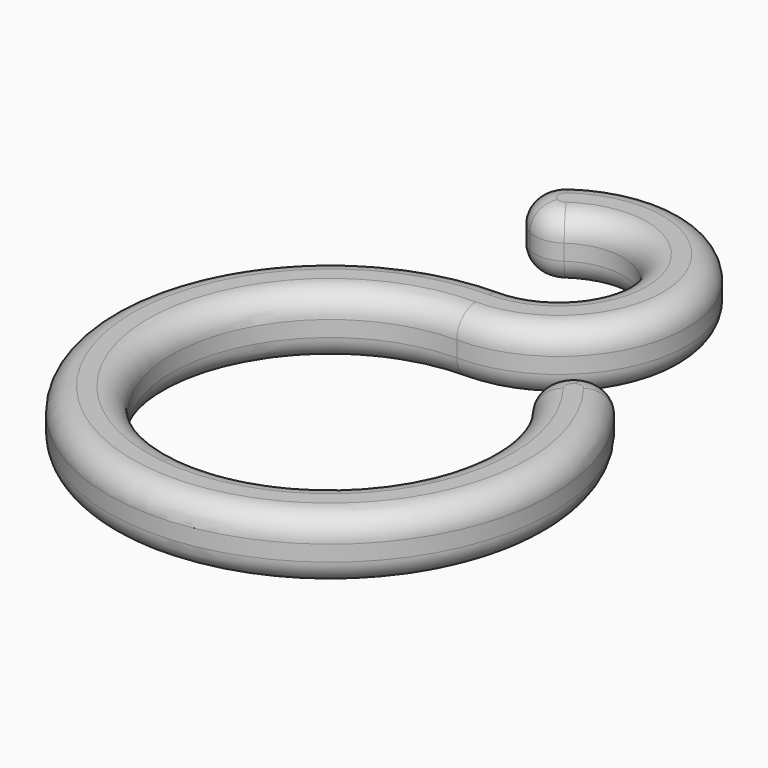
from build123d import *

# Parameters (mm, degrees)
F1_DEPTH = 4
F2_R     = 1.99999
F3_R     = 1.5


# Not quite as in the source:
# - a fillet or chamfer is up to 0.001 mm smaller than in the source, because OpenCascade refuses the exact size


with BuildPart() as f1:
    # F0 (on Top) → F1 (new body)
    with BuildSketch(Plane.XY):
        with BuildLine():
            ThreePointArc((-6.4063729182, 27.757124237), (0.3935028475, 26.9429632102), (-3.2635407988, 21.152695481))
            ThreePointArc((-3.2635407988, 21.152695481), (-8.7172147503, -5.7413900015), (6.782193219, 16.9037583997))
            Line((6.782193219, 16.9037583997), (2.7912945952, 15.1112737681))
            ThreePointArc((2.7912945952, 15.1112737681), (-6.4583973785, -2.3232156327), (-3.2635407988, 17.152695481))
            ThreePointArc((-3.2635407988, 17.152695481), (3.8117374796, 29.0423487575), (-10.0130104693, 29.5898539199))
            Line((-10.0130104693, 29.5898539199), (-6.4063729182, 27.757124237))
        make_face()
    extrude(amount=F1_DEPTH)

    # F2 (radius 2 in the source; OpenCascade refuses exactly that, so slightly less here)
    f2_edges = [f1.edges().sort_by_distance(p)[0] for p in [
        (-10.01301, 29.589854, 2),
        (-6.406373, 27.757124, 2),
        (2.791295, 15.111274, 2),
        (6.782193, 16.903758, 2),
    ]]
    fillet(f2_edges, radius=F2_R)

    # F3
    f3_edges = [f1.edges().sort_by_distance(p)[0] for p in [
        (-9.447025, -5.407739, 4),
        (-9.447025, -5.407739, 0),
    ]]
    fillet(f3_edges, radius=F3_R)


solid = f1.part
